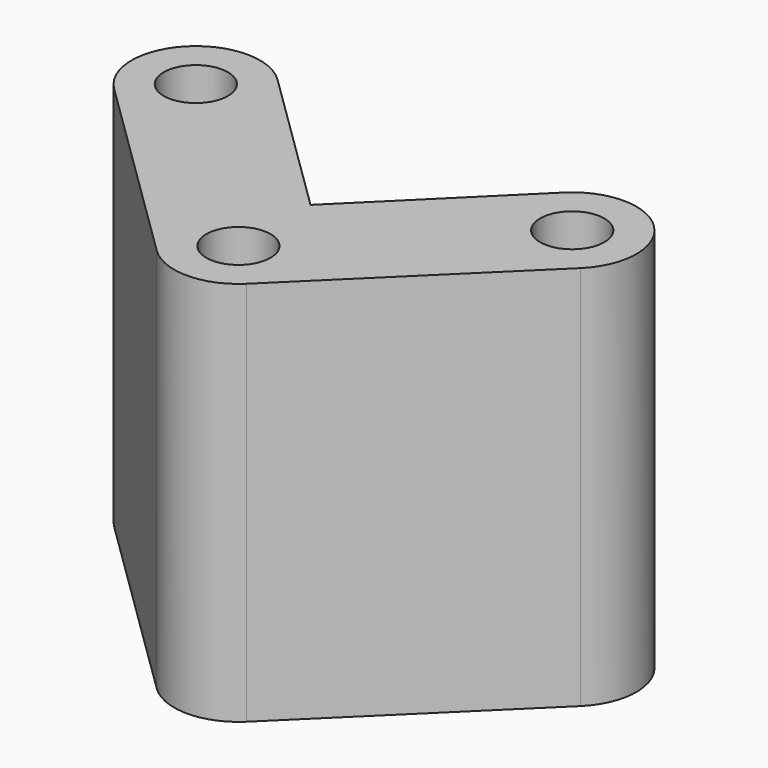
from build123d import *

# Parameters (mm, degrees)
F0_R     = 12.5
F1_DEPTH = 150
F3_DEPTH = 50


# Not quite as in the source:
# - the program builds the solid bodies; features that only make, move or delete a surface that nothing else refers to are left out


with BuildPart() as f1:
    # F0 (on Top) → F1 (new body)
    with BuildSketch(Plane.XY):
        with BuildLine():
            Line((8.6845052377, -18.7444362128), (-50.6748429861, 39.3975202147))
            ThreePointArc((-50.6748429861, 39.3975202147), (-86.0282846169, 39.0312350068), (-85.661999409, 3.6777933759))
            Line((-85.661999409, 3.6777933759), (-9.0315715293, -71.3810327757))
            ThreePointArc((-9.0315715293, -71.3810327757), (8.4718011348, -78.5211674377), (25.9695737293, -71.3673200922))
            Line((25.9695737293, -71.3673200922), (98.7170861934, 0))
            ThreePointArc((98.7170861934, 0), (99.0182133881, 35.3918171352), (63.6258335307, 35.6173071466))
            Line((63.6258335307, 35.6173071466), (8.6845052377, -18.7444362128))
        make_face()
        with Locations((8.4620066821, -53.5211693563)):
            Circle(F0_R, mode=Mode.SUBTRACT)
        with Locations((-68.1684211975, 21.5376567953)):
            Circle(F0_R, mode=Mode.SUBTRACT)
        with Locations((81.2095191462, 17.8461507359)):
            Circle(F0_R, mode=Mode.SUBTRACT)
    extrude(amount=F1_DEPTH)

    # F0 (on Top) → F3 (join)
    with BuildSketch(Plane.XY):
        with BuildLine():
            Line((8.6845052377, -18.7444362128), (-50.6748429861, 39.3975202147))
            ThreePointArc((-50.6748429861, 39.3975202147), (-86.0282846169, 39.0312350068), (-85.661999409, 3.6777933759))
            Line((-85.661999409, 3.6777933759), (-9.0315715293, -71.3810327757))
            ThreePointArc((-9.0315715293, -71.3810327757), (8.4718011348, -78.5211674377), (25.9695737293, -71.3673200922))
            Line((25.9695737293, -71.3673200922), (98.7170861934, 0))
            ThreePointArc((98.7170861934, 0), (99.0182133881, 35.3918171352), (63.6258335307, 35.6173071466))
            Line((63.6258335307, 35.6173071466), (8.6845052377, -18.7444362128))
        make_face()
        with Locations((8.4620066821, -53.5211693563)):
            Circle(F0_R, mode=Mode.SUBTRACT)
        with Locations((-68.1684211975, 21.5376567953)):
            Circle(F0_R, mode=Mode.SUBTRACT)
        with Locations((81.2095191462, 17.8461507359)):
            Circle(F0_R, mode=Mode.SUBTRACT)
    extrude(amount=F3_DEPTH)


solid = f1.part
